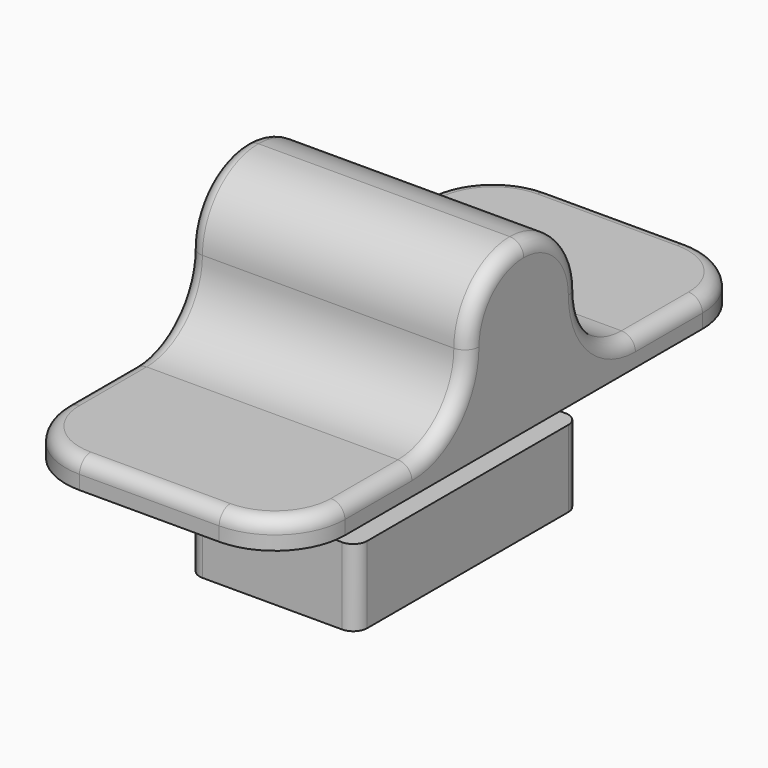
from build123d import *

# Parameters (mm, degrees)
F0_W      = 20
F0_H      = 42
F1_DEPTH  = 2
F2_W      = 12
F2_H      = 20
F3_DEPTH  = 10
F4_R      = 1
F5_W      = 20
F5_H      = 10
F6_DEPTH  = 10
F7_R      = 4.99999
F8_R      = 3.6
F9_DEPTH  = 8
F10_W     = 2
F10_H     = 5
F11_DEPTH = 7
F12_R     = 5
F13_W     = 25
F13_H     = 2
F14_DEPTH = 2
F15_W     = 28.3062260176
F15_H     = 2
F16_DEPTH = 2
F17_R     = 1


# Not quite as in the source:
# - a fillet or chamfer is up to 0.001 mm smaller than in the source, because OpenCascade refuses the exact size


with BuildPart() as f1:
    # F0 (on Top) → F1 (new body)
    with BuildSketch(Plane.XY):
        Rectangle(F0_W, F0_H)
    extrude(amount=F1_DEPTH)

    # F2 (on Top) → F3 (join)
    with BuildSketch(Plane.XY):
        Rectangle(F2_W, F2_H)
    extrude(amount=-F3_DEPTH)

    # F4
    f4_edges = [f1.edges().sort_by_distance(p)[0] for p in [
        (-6, -10, -5),
        (6, -10, -5),
        (-6, 10, -5),
        (6, 10, -5),
    ]]
    fillet(f4_edges, radius=F4_R)

    # F5 (on face) → F6 (join)
    with BuildSketch(Plane.XY.offset(2)):
        Rectangle(F5_W, F5_H)
    extrude(amount=F6_DEPTH)

    # F7 (radius 5 in the source; OpenCascade refuses exactly that, so slightly less here)
    f7_edges = [f1.edges().sort_by_distance(p)[0] for p in [
        (0, -5, 12),
        (0, 5, 12),
        (0, -5, 2),
        (0, 5, 2),
    ]]
    fillet(f7_edges, radius=F7_R)

    # F8 (on face) → F9 (cut)
    with BuildSketch(Plane(origin=(0, 0, -10), x_dir=(1, 0, 0), z_dir=(0, 0, -1))):
        Circle(F8_R)
    extrude(amount=-F9_DEPTH, mode=Mode.SUBTRACT)

    # F10 (on face) → F11 (cut)
    with BuildSketch(Plane(origin=(0, 10, 0), x_dir=(-1, 0, 0), z_dir=(0, 1, 0))):
        with Locations((0, -7.5)):
            Rectangle(F10_W, F10_H)
    extrude(amount=-F11_DEPTH, mode=Mode.SUBTRACT)

    # F12
    f12_edges = [f1.edges().sort_by_distance(p)[0] for p in [
        (10, -21, 1),
        (-10, 21, 1),
        (10, 21, 1),
        (-10, -21, 1),
    ]]
    fillet(f12_edges, radius=F12_R)

    # F13 (on face) → F14 (cut)
    with BuildSketch(Plane(origin=(-6, 0, 0), x_dir=(0, -1, 0), z_dir=(-1, 0, 0))):
        with Locations((-0.9450479232, -3.5)):
            Rectangle(F13_W, F13_H)
    extrude(amount=-F14_DEPTH, mode=Mode.SUBTRACT)

    # F15 (on face) → F16 (cut)
    with BuildSketch(Plane.YZ.offset(6)):
        with Locations((-0.2904124558, -3.5)):
            Rectangle(F15_W, F15_H)
    extrude(amount=-F16_DEPTH, mode=Mode.SUBTRACT)

    # F17
    f17_edges = [f1.edges().sort_by_distance(p)[0] for p in [
        (-10, -3.535537, 10.535537),
    ]]
    fillet(f17_edges, radius=F17_R)


solid = f1.part
